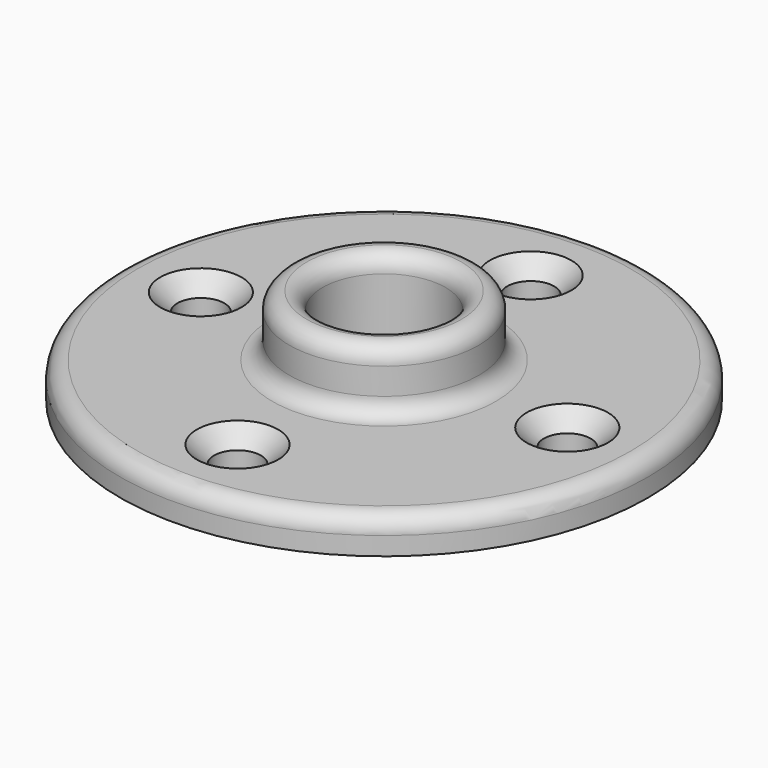
from build123d import *

# Parameters (mm, degrees)
F0_R     = 38.9255
F0_R_2   = 3.46075
F0_R_3   = 13.97
F1_DEPTH = 5.2324
F0_R_4   = 9.0805
F2_DEPTH = 14.224
F3_R     = 2.54
F5_SIZE  = 2.54


# Not quite as in the source:
# - a fillet or chamfer that OpenCascade refuses, or shapes differently, is made with other operations: its cross-section is extruded or revolved along the edge and cut away or added


with BuildPart() as f1:
    # F0 (on Top) → F1 (new body)
    with BuildSketch(Plane.XY):
        Circle(F0_R)
        with Locations((0, -27.01925)):
            Circle(F0_R_2, mode=Mode.SUBTRACT)
        with Locations((-27.01925, 0)):
            Circle(F0_R_2, mode=Mode.SUBTRACT)
        Circle(F0_R_3, mode=Mode.SUBTRACT)
        with Locations((27.01925, 0)):
            Circle(F0_R_2, mode=Mode.SUBTRACT)
        with Locations((0, 27.01925)):
            Circle(F0_R_2, mode=Mode.SUBTRACT)
    extrude(amount=F1_DEPTH)

    # F0 (on Top) → F2 (join)
    with BuildSketch(Plane.XY):
        Circle(F0_R_3)
        Circle(F0_R_4, mode=Mode.SUBTRACT)
    extrude(amount=F2_DEPTH)

    # F3
    f3_edges = [f1.edges().sort_by_distance(p)[0] for p in [
        (-38.9255, 0, 5.2324),
        (-13.97, 0, 14.224),
        (-13.97, 0, 5.2324),
    ]]
    fillet(f3_edges, radius=F3_R)

    # F4: fillet of radius 2.54 on 1 edges, made by hand

    # F4_s1 → F4_t2 (revolve, cut)
    with BuildSketch(Plane.XZ):
        with BuildLine():
            ThreePointArc((9.0805, 11.6911538243), (9.7583144561, 13.4185405789), (11.43, 14.224))
            Line((11.43, 14.224), (9.0805, 14.224))
            Line((9.0805, 14.224), (9.0805, 11.6911538243))
        make_face()
    revolve(axis=Axis((0, 0, 14.224), (0, 0, 1)), mode=Mode.SUBTRACT)

    # F5
    f5_edges = [f1.edges().sort_by_distance(p)[0] for p in [
        (-3.46075, 27.01925, 5.2324),
        (23.5585, 0, 5.2324),
        (-3.46075, -27.01925, 5.2324),
        (-30.48, 0, 5.2324),
    ]]
    chamfer(f5_edges, length=F5_SIZE)


solid = f1.part
